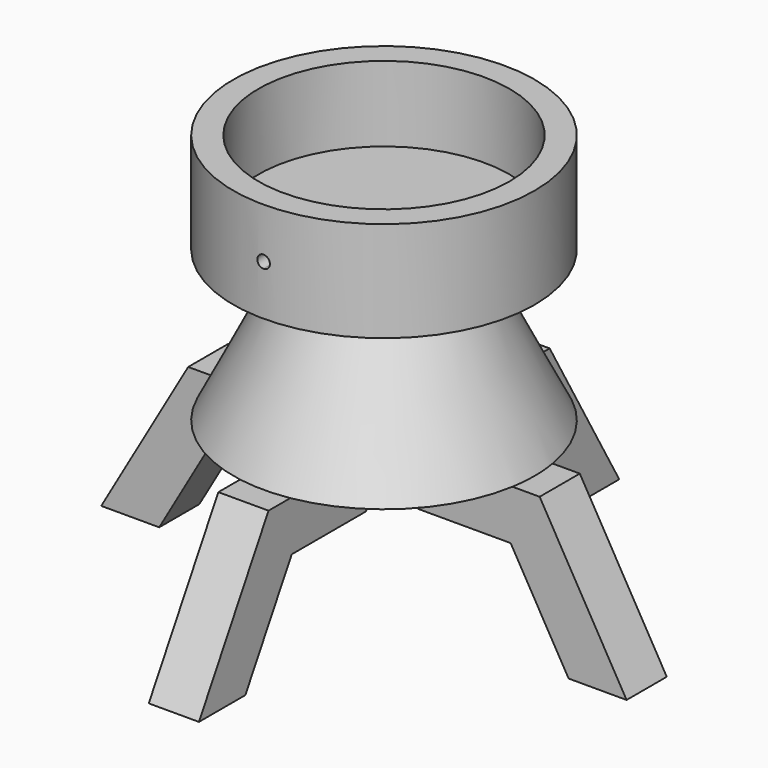
from build123d import *

# Parameters (mm, degrees)
F2_DEPTH  = 25.4
F3_DEPTH  = 25.4
F4_R      = 152.4
F6_R      = 76.2
F8_R      = 152.4
F8_R_2    = 76.2
F9_DEPTH  = 101.6
F10_R     = 127
F11_DEPTH = 76.2
F13_DEPTH = 265.7891810245


with BuildPart() as f2:
    # F0 (on Front) → F2 (new body, symmetric)
    with BuildSketch(Plane.XZ):
        Polygon((177.8, 0), (25.4, 0), (54.7293936748, -50.8), (148.4706063252, -50.8), (177.8, -50.8), align=None)
        Polygon((207.1293936748, -50.8), (177.8, 0), (177.8, -50.8), align=None)
        Polygon((177.8, -50.8), (148.4706063252, -50.8), (177.8, -101.6), align=None)
        Polygon((207.1293936748, -50.8), (177.8, -50.8), (177.8, -101.6), (207.1293936748, -152.4), (265.7881810245, -152.4), align=None)
    extrude(amount=F2_DEPTH, both=True)



with BuildPart() as f2b:
    # F0 (on Front) → F2, piece 2 (new body, symmetric)
    with BuildSketch(Plane.XZ):
        Polygon((-54.7293936748, -50.8), (-25.4, 0), (-177.8, 0), (-207.1293936748, -50.8), (-148.4706063252, -50.8), align=None)
        Polygon((-207.1293936748, -152.4), (-148.4706063252, -50.8), (-207.1293936748, -50.8), (-265.7881810245, -152.4), align=None)
    extrude(amount=F2_DEPTH, both=True)


with BuildPart() as f2_1:
    add(f2.part)

    add(f2b.part)  # F3 merges F2b
    # F1 (on Right) → F3 (join, symmetric)
    with BuildSketch(Plane.YZ):
        Polygon((177.8, 0), (25.4, 0), (54.7293936748, -50.8), (148.4706063252, -50.8), (177.8, -50.8), align=None)
        Polygon((-54.7293936748, -50.8), (-25.4, 0), (-177.8, 0), (-207.1293936748, -50.8), (-148.4706063252, -50.8), align=None)
        Polygon((207.1293936748, -50.8), (177.8, 0), (177.8, -50.8), align=None)
        Polygon((177.8, -50.8), (148.4706063252, -50.8), (177.8, -101.6), align=None)
        Polygon((207.1293936748, -50.8), (177.8, -50.8), (177.8, -101.6), (207.1293936748, -152.4), (222.5192777686, -152.4), (265.7881810245, -152.4), align=None)
        Polygon((-207.1293936748, -152.4), (-148.4706063252, -50.8), (-207.1293936748, -50.8), (-265.7881810245, -152.4), align=None)
    extrude(amount=F3_DEPTH, both=True)

    # F4 (on Top) → F7 section 0
    with BuildSketch(Plane.XY):
        Circle(F4_R)
    # F6 (on offset) → F7 section 1
    with BuildSketch(Plane.XY.offset(152.4)):
        Circle(F6_R)
    loft()

    # F8 (on face) → F9 (join)
    with BuildSketch(Plane.XY.offset(152.4)):
        Circle(F8_R)
        Circle(F8_R_2, mode=Mode.SUBTRACT)
        Circle(F8_R_2)
    extrude(amount=F9_DEPTH)

    # F10 (on face) → F11 (cut)
    with BuildSketch(Plane.XY.offset(254)):
        Circle(F10_R)
    extrude(amount=-F11_DEPTH, mode=Mode.SUBTRACT)

    # F12 (on Front) → F13 (cut, through all)
    with BuildSketch(Plane.XZ):
        with BuildLine():
            ThreePointArc((0, 196.85), (4.4901280605, 198.7098719395), (6.35, 203.2))
            ThreePointArc((6.35, 203.2), (-4.4901280605, 207.6901280605), (0, 196.85))
        make_face()
    extrude(amount=F13_DEPTH, mode=Mode.SUBTRACT)


solid = f2_1.part
